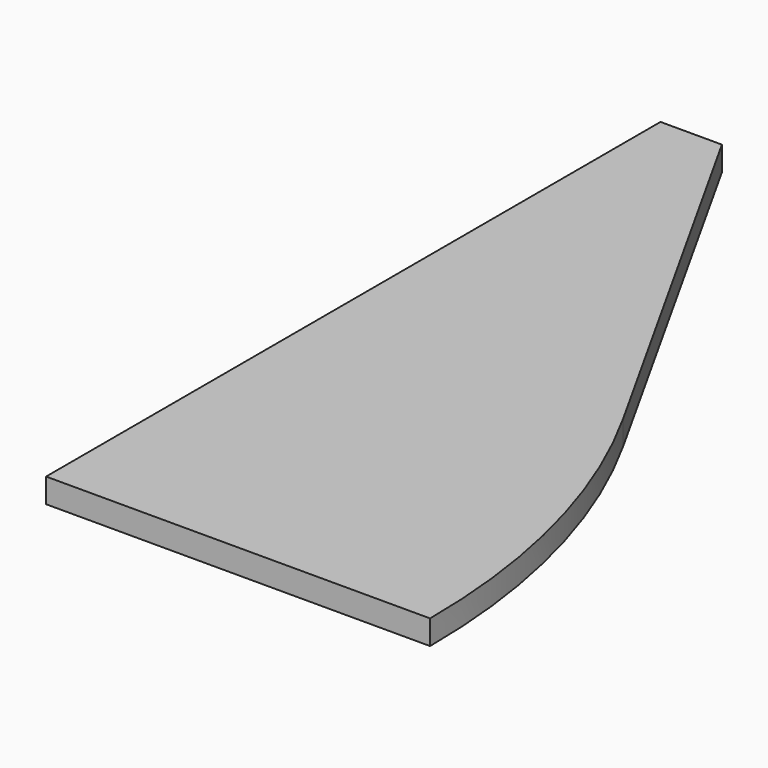
from build123d import *

# Parameters (mm, degrees)
F1_DEPTH = 3.175


# Not quite as in the source:
# - a length typed as a fraction of an inch, garbled in the dataset ("3 / 203.2 mm" for 3/8 in), is restored


with BuildPart() as f1:
    # F0 (on Top) → F1 (new body)
    with BuildSketch(Plane.XY):
        with BuildLine():
            Line((-25, -50), (25, -50))
            ThreePointArc((25, -50), (21.9136795769, -25.9174991328), (12.8542008758, -3.3915570341))
            Line((12.8542008758, -3.3915570341), (-17, 50))
            Line((-17, 50), (-25, 50))
            Line((-25, 50), (-25, -50))
        make_face()
    extrude(amount=F1_DEPTH)


solid = f1.part
